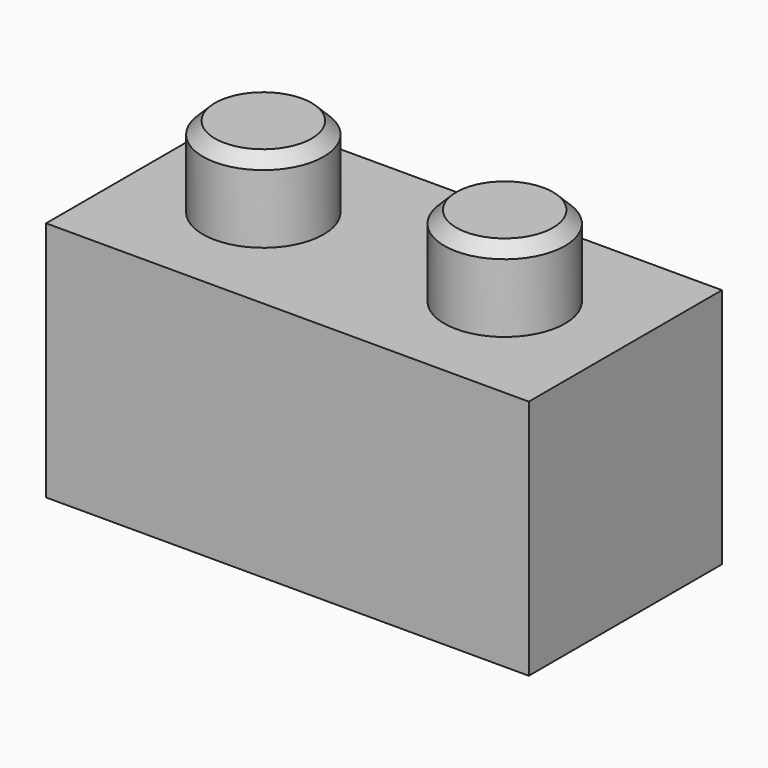
from build123d import *

# Parameters (mm, degrees)
F3_W     = 12
F3_H     = 6
F0_DEPTH = 6.0000000522
F1_R     = 1.5
F4_DEPTH = 2
F5_SIZE  = 0.3
F2_T     = 1


# Not quite as in the source:
# - a shell that OpenCascade refuses in one call is made with other operations: the cavity is built on its own and cut out


with BuildPart() as f0:
    # F3 (on Top) → F0 (new body)
    with BuildSketch(Plane.XY):
        Rectangle(F3_W, F3_H)
    extrude(amount=-F0_DEPTH)

    # F1 (on Top) → F4 (join)
    with BuildSketch(Plane.XY):
        with Locations((3, 0)):
            Circle(F1_R)
        with Locations((-3, 0)):
            Circle(F1_R)
    extrude(amount=F4_DEPTH)

    # F5
    f5_edges = [f0.edges().sort_by_distance(p)[0] for p in [
        (-4.5, 0, 2),
        (1.5, 0, 2),
    ]]
    chamfer(f5_edges, length=F5_SIZE)

    # F2: shell of thickness 1, made by hand


with BuildPart() as f2_core1:
    # F2_t2: copy of F0
    add(f0.part)

    # the walls: a layer under each face that stays
    f2_faces = [f2_core1.faces().sort_by_distance(p)[0] for p in [
        (-4.5, 0, 0.85),
        (-4.35, 0, 1.85),
        (0, 0, 0),
        (-3, 0, 2),
        (0, 3, -3.0000000261),
        (6, 0, -3.0000000261),
        (-6, 0, -3.0000000261),
        (0, -3, -3.0000000261),
        (1.5, 0, 0.85),
        (1.65, 0, 1.85),
        (3, 0, 2),
    ]]
    thicken(f2_faces, amount=-F2_T, mode=Mode.SUBTRACT)

    # F2_s3 → F2_t4 (revolve, cut)
    with BuildSketch(Plane.XZ):
        Polygon((-1.49, 0.01), (-2.5, 0), (-2.5, -1), (-1.5, -1), align=None)
    revolve(axis=Axis((-3, 0, 0), (0, 0, 1)), mode=Mode.SUBTRACT)

    # F2_s5 → F2_t6 (revolve, cut)
    with BuildSketch(Plane.XZ):
        Polygon((4.51, 0.01), (4.5, -1), (3.5, -1), (3.5, 0), align=None)
    revolve(axis=Axis((3, 0, 0), (0, 0, 1)), mode=Mode.SUBTRACT)


with BuildPart() as f0_1:
    add(f0.part)

    # what is left inside the walls is the cavity
    f2_cavity = [f2_core1.part.solids().sort_by_distance(p)[0] for p in [
        (0, 1.99, -4.333333),
    ]]
    add(f2_cavity, mode=Mode.SUBTRACT)


solid = f0_1.part
